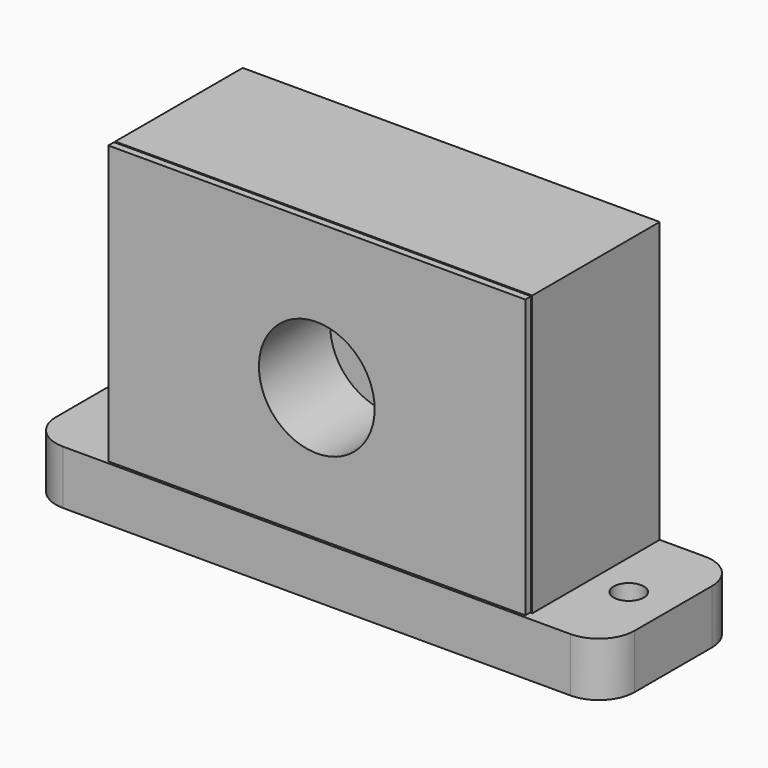
from build123d import *

# Parameters (mm, degrees)
F0_W      = 59.5
F0_H      = 41.5
F0_R      = 6
F0_R_2    = 11.5
F1_DEPTH  = 21.5
F7_W      = 38.354
F7_H      = 38.354
F8_DEPTH  = 19.05
F9_W      = 11.303
F9_H      = 5.588
F10_DEPTH = 2.451
F12_D     = 2.9464
F13_W     = 23.974
F13_H     = 7.718
F13_W_2   = 20.828
F13_H_2   = 4.572
F14_DEPTH = 59.5
F15_DEPTH = 1.237
F16_W     = 5.493
F16_H     = 24.687
F17_DEPTH = 17.78
F18_W     = 37.846
F18_H     = 37.846
F18_R     = 8.255
F19_DEPTH = 12.7
F20_W     = 59.5
F20_H     = 39.673
F20_R     = 8.255
F21_DEPTH = 1.016
F22_W     = 23.974
F22_H     = 7.718
F23_DEPTH = 41.275
F24_R     = 2.159
F25_DEPTH = 25.4
F26_R     = 5.08


# Not quite as in the source:
# - a feature of the source that left no trace in its solid (it failed there, or was rolled back) is left out
# - a pattern or mirror of a feature is missing from the dataset's text; its kind, count and spacing are read off the source's solid


with BuildPart() as f1:
    # F0 (on Front) → F1 (new body)
    with BuildSketch(Plane.XZ):
        Rectangle(F0_W, F0_H)
        with Locations((-17.25, -10.75)):
            Circle(F0_R, mode=Mode.SUBTRACT)
        with BuildLine():
            ThreePointArc((-23.75, 14.75), (-23.4571067812, 15.4571067812), (-22.75, 15.75))
            Line((-22.75, 15.75), (-11.25, 15.75))
            ThreePointArc((-11.25, 15.75), (-10.5428932188, 15.4571067812), (-10.25, 14.75))
            Line((-10.25, 14.75), (-10.25, -0.25))
            ThreePointArc((-10.25, -0.25), (-10.5428932188, -0.9571067812), (-11.25, -1.25))
            Line((-11.25, -1.25), (-22.75, -1.25))
            ThreePointArc((-22.75, -1.25), (-23.4571067812, -0.9571067812), (-23.75, -0.25))
            Line((-23.75, -0.25), (-23.75, 14.75))
        make_face(mode=Mode.SUBTRACT)
        with Locations((14.45, 7.05)):
            Circle(F0_R_2, mode=Mode.SUBTRACT)
        with BuildLine():
            Line((-11.25, 15.75), (-22.75, 15.75))
            ThreePointArc((-22.75, 15.75), (-23.4571067812, 15.4571067812), (-23.75, 14.75))
            Line((-23.75, 14.75), (-23.75, -0.25))
            ThreePointArc((-23.75, -0.25), (-23.4571067812, -0.9571067812), (-22.75, -1.25))
            Line((-22.75, -1.25), (-11.25, -1.25))
            ThreePointArc((-11.25, -1.25), (-10.5428932188, -0.9571067812), (-10.25, -0.25))
            Line((-10.25, -0.25), (-10.25, 14.75))
            ThreePointArc((-10.25, 14.75), (-10.5428932188, 15.4571067812), (-11.25, 15.75))
        make_face()
        with Locations((14.45, 7.05)):
            Circle(F0_R_2)
        with Locations((-17.25, -10.75)):
            Circle(F0_R)
    extrude(amount=-F1_DEPTH)

    # F7 (on face) → F8 (cut)
    with BuildSketch(Plane.XZ):
        Rectangle(F7_W, F7_H)
    extrude(amount=-F8_DEPTH, mode=Mode.SUBTRACT)

    # F9 (on face) → F10 (cut, through all)
    with BuildSketch(Plane.XZ.offset(-19.05)):
        with Locations((4.8895, -13.208)):
            Rectangle(F9_W, F9_H)
    extrude(amount=-F10_DEPTH, mode=Mode.SUBTRACT)

    # F12 (through all)
    with Locations(Plane.XZ.offset(-19.05)):
        with Locations((-13.97, 13.97), (13.97, 13.97), (13.97, -13.97), (-13.97, -13.97)):
            Hole(F12_D / 2)

    # F13 (on face) → F14 (join, through all)
    with BuildSketch(Plane.YZ.offset(29.75)):
        with Locations((10.75, -23.036)):
            Rectangle(F13_W, F13_H)
        with Locations((10.75, -23.036)):
            Rectangle(F13_W_2, F13_H_2, mode=Mode.SUBTRACT)
    extrude(amount=-F14_DEPTH)

    # F15 (add, through all): a face of the model
    f15_faces = [f1.faces().sort_by_distance(p)[0] for p in [
        (-0.1351406862, 21.5, 1.1826798979),
    ]]
    extrude(f15_faces, amount=F15_DEPTH)

    # F16 (on face) → F17 (cut)
    with BuildSketch(Plane.XZ):
        with Locations((-24.4635, 0.7865)):
            Rectangle(F16_W, F16_H)
    f17 = extrude(amount=-F17_DEPTH, mode=Mode.SUBTRACT)

    # F17_copies: F17 across plane
    add(f17.mirror(Plane(origin=(0, 0, 0), x_dir=(0, 0, 1), z_dir=(1, 0, 0))), mode=Mode.SUBTRACT)

    # F22 (on Right) → F23 (join, symmetric)
    with BuildSketch(Plane.YZ):
        with Locations((10.75, -23.036)):
            Rectangle(F22_W, F22_H)
    extrude(amount=F23_DEPTH, both=True)

    # F24 (on face) → F25 (cut)
    with BuildSketch(Plane(origin=(0, 0, -26.895), x_dir=(1, 0, 0), z_dir=(0, 0, -1))):
        with Locations((-34.925, -10.75)):
            Circle(F24_R)
        with Locations((34.925, -10.75)):
            Circle(F24_R)
    extrude(amount=-F25_DEPTH, mode=Mode.SUBTRACT)

    # F26
    f26_edges = [f1.edges().sort_by_distance(p)[0] for p in [
        (-41.275, 22.737, -23.036),
        (-41.275, -1.237, -23.036),
        (41.275, 22.737, -23.036),
        (41.275, -1.237, -23.036),
    ]]
    fillet(f26_edges, radius=F26_R)


with BuildPart() as f19:
    # F18 (on face) → F19 (new body)
    with BuildSketch(Plane.XZ.offset(1.237)):
        Rectangle(F18_W, F18_H)
        Circle(F18_R, mode=Mode.SUBTRACT)
    extrude(amount=-F19_DEPTH)

    # F20 (on face) → F21 (join)
    with BuildSketch(Plane.XZ.offset(1.237)):
        with Locations((0, 0.9135)):
            Rectangle(F20_W, F20_H)
        Circle(F20_R, mode=Mode.SUBTRACT)
    extrude(amount=-F21_DEPTH)


solid = Compound([f1.part, f19.part])
